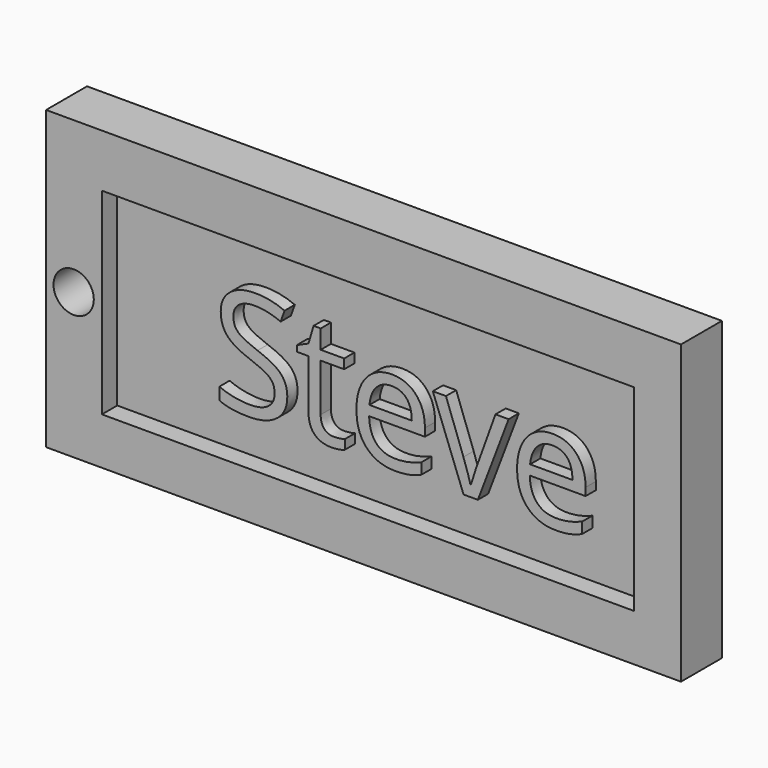
from build123d import *

# Parameters (mm, degrees)
F0_W         = 63.0088448524
F0_H         = 29.4643603265
F0_W_2       = 52.8024672531
F0_H_2       = 19.5456631482
F1_DEPTH     = 5.08
F2_DEPTH     = 3.175
F4_TEXT_SIZE = 15.0147783251
F5_DEPTH     = 1.27
F3_R         = 1.9991797934
F6_DEPTH     = 25.4


# Not quite as in the source:
# - Text() gives the source's letters only with a copy of the font that has no kerning and outlines rounded to 1/6400 em; it was checked with that copy


with BuildPart() as f1:
    # F0 (on Front) → F1 (new body)
    with BuildSketch(Plane.XZ):
        with Locations((31.5044224262, 19.3307865411)):
            Rectangle(F0_W, F0_H)
        with Locations((31.9399938453, 19.0390590578)):
            Rectangle(F0_W_2, F0_H_2, mode=Mode.SUBTRACT)
    extrude(amount=F1_DEPTH)

    # F0 (on Front) → F2 (join)
    with BuildSketch(Plane.XZ):
        with Locations((31.9399938453, 19.0390590578)):
            Rectangle(F0_W_2, F0_H_2)
    extrude(amount=F2_DEPTH)

    # F4 (on face) → F5 (join)
    with BuildSketch(Plane.XZ.offset(3.175)):
        with Locations((15.9080849125, 13.5122802191)):
            Text('Steve', F4_TEXT_SIZE, font='Open Sans', text_align=(TextAlign.LEFT, TextAlign.BOTTOM))
    extrude(amount=F5_DEPTH)

    # F3 (on face) → F6 (cut)
    with BuildSketch(Plane.XZ.offset(5.08)):
        with Locations((2.7384241112, 19.0390590578)):
            Circle(F3_R)
    extrude(amount=-F6_DEPTH, mode=Mode.SUBTRACT)


solid = f1.part
